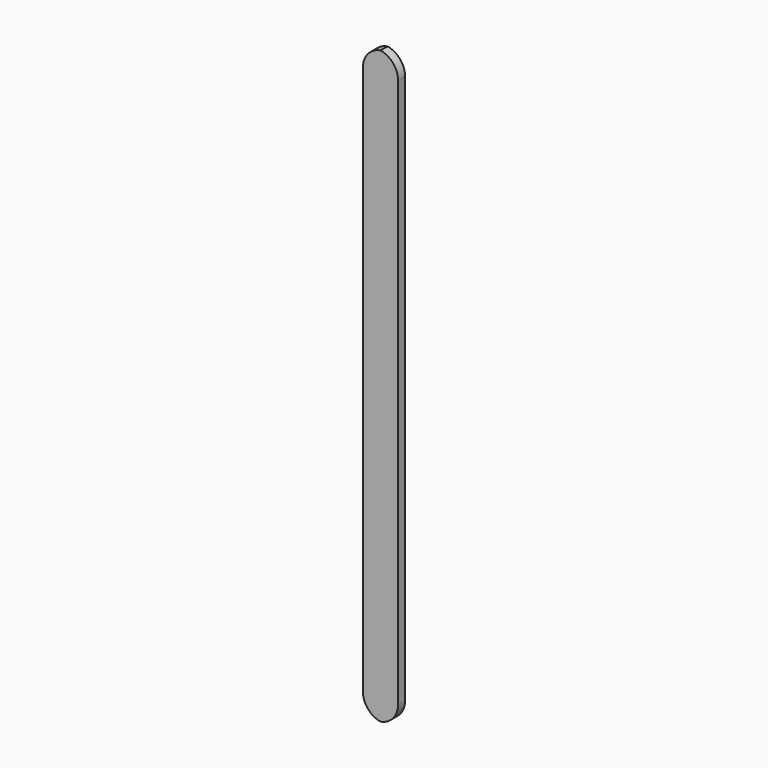
from build123d import *

# Parameters (mm, degrees)
F0_W        = 6.35
F0_H        = 106.68
F1_DEPTH    = 1.5875
F2_T1_DEPTH = 20.6375
F3_T1_DEPTH = 20.6375


# Not quite as in the source:
# - a fillet or chamfer that OpenCascade refuses, or shapes differently, is made with other operations: its cross-section is extruded or revolved along the edge and cut away or added


with BuildPart() as f1:
    # F0 (on Front) → F1 (new body)
    with BuildSketch(Plane.XZ):
        with Locations((-32.9172081137, -12.1981453611)):
            Rectangle(F0_W, F0_H)
    extrude(amount=F1_DEPTH)

    # F2: fillet of radius 3.81 on 2 edges, made by hand

    # F2_s2 → F2_t1 (cut)
    with BuildSketch(Plane.XZ.offset(-9.525)):
        with BuildLine():
            ThreePointArc((-36.0922081137, 37.3318546389), (-34.97628495, 40.0259314752), (-32.2822081137, 41.1418546389))
            Line((-32.2822081137, 41.1418546389), (-36.0922081137, 41.1418546389))
            Line((-36.0922081137, 41.1418546389), (-36.0922081137, 37.3318546389))
        make_face()
        with BuildLine():
            ThreePointArc((-29.7422081137, 37.3318546389), (-30.8581312774, 40.0259314752), (-33.5522081137, 41.1418546389))
            Line((-33.5522081137, 41.1418546389), (-29.7422081137, 41.1418546389))
            Line((-29.7422081137, 41.1418546389), (-29.7422081137, 37.3318546389))
        make_face()
    extrude(amount=F2_T1_DEPTH, mode=Mode.SUBTRACT)

    # F3: fillet of radius 3.81 on 2 edges, made by hand

    # F3_s2 → F3_t1 (cut)
    with BuildSketch(Plane.XZ.offset(-9.525)):
        with BuildLine():
            ThreePointArc((-36.0922081137, -61.7281453611), (-34.97628495, -64.4222221974), (-32.2822081137, -65.5381453611))
            Line((-32.2822081137, -65.5381453611), (-36.0922081137, -65.5381453611))
            Line((-36.0922081137, -65.5381453611), (-36.0922081137, -61.7281453611))
        make_face()
        with BuildLine():
            ThreePointArc((-33.5522081137, -65.5381453611), (-30.8581312774, -64.4222221974), (-29.7422081137, -61.7281453611))
            Line((-29.7422081137, -61.7281453611), (-29.7422081137, -65.5381453611))
            Line((-29.7422081137, -65.5381453611), (-33.5522081137, -65.5381453611))
        make_face()
    extrude(amount=F3_T1_DEPTH, mode=Mode.SUBTRACT)


solid = f1.part
